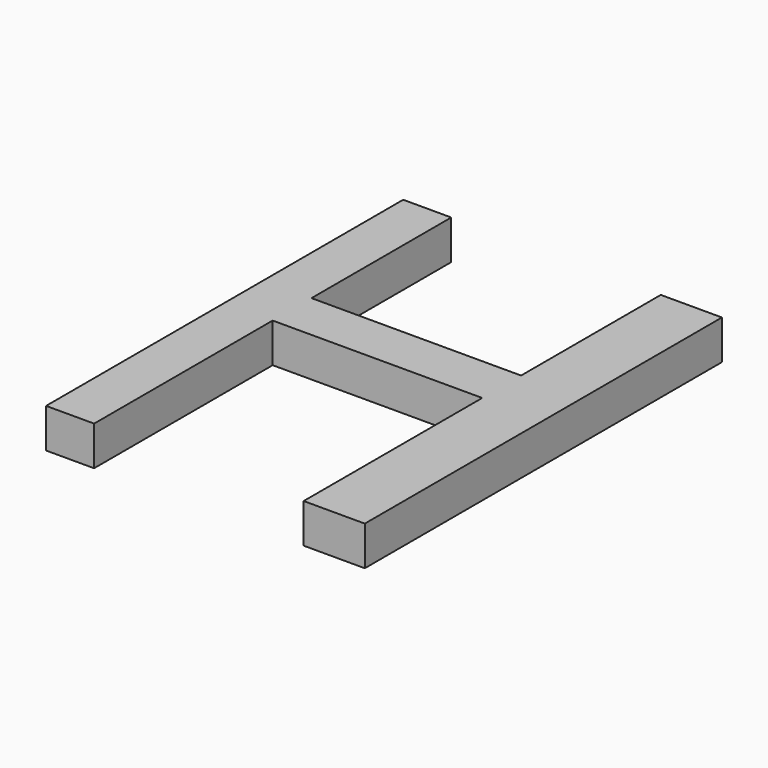
from build123d import *

# Parameters (mm, degrees)
F0_W     = 67.6902830601
F0_H     = 15.6858190894
F1_DEPTH = 12.7


with BuildPart() as f1:
    # F0 (on Top) → F1 (new body)
    with BuildSketch(Plane.XY):
        Polygon((-369.42923069, 144.1887915134), (-384.9415779114, 144.1887915134), (-384.9415779114, 0), (-369.42923069, 0), (-369.42923069, 72.0943957567), (-369.42923069, 87.7802148461), align=None)
        with Locations((-335.58408916, 79.9373053014)):
            Rectangle(F0_W, F0_H)
        Polygon((-301.7389476299, 144.1887915134), (-301.7389476299, 87.7802148461), (-301.7389476299, 72.0943957567), (-301.7389476299, 0), (-281.995922327, 0), (-281.995922327, 144.1887915134), align=None)
    extrude(amount=F1_DEPTH)


solid = f1.part
